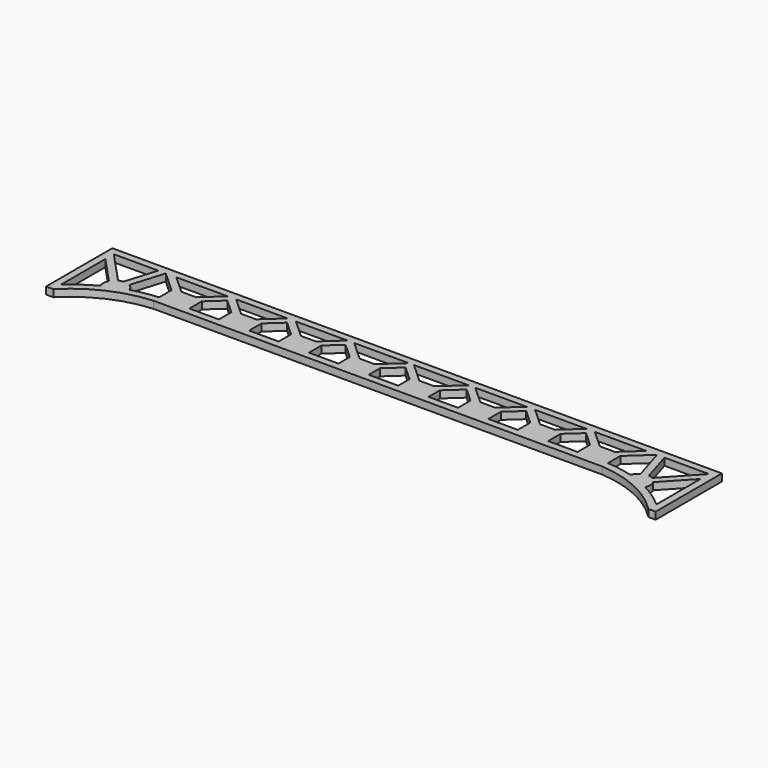
from build123d import *

# Parameters (mm, degrees)
F1_DEPTH = 1


# Not quite as in the source:
# - ends of sketch curves that miss each other by under 0.0002 mm in the source are joined


with BuildPart() as f1:
    # F0 (on Top) → F1 (new body)
    with BuildSketch(Plane.XY):
        with BuildLine():
            ThreePointArc((31.2898730428, -1.0903693776), (36.8162528215, -2.4992396802), (41.4861883055, -5.7729976987))
            Line((41.4861883055, -5.7729976987), (42.499983, -5.772998))
            Line((42.499983, -5.772998), (42.499983, 5.772998))
            Line((42.499983, 5.772998), (-42.499983, 5.772998))
            Line((-42.499983, 5.772998), (-42.499983, -5.772998))
            Line((-42.499983, -5.772998), (-41.486188, -5.772998))
            ThreePointArc((-41.486188, -5.772998), (-36.8162528215, -2.4992396802), (-31.2898730428, -1.0903693776))
            Line((-31.2898730428, -1.0903693776), (31.2898730428, -1.0903693776))
        make_face()
        with BuildLine():
            ThreePointArc((-37.980823226, -1.9562535657), (-39.8184929613, -3.0669655752), (-41.4999834083, -4.4023685483))
            Line((-41.4999834083, -4.4023685483), (-41.499983, 3.305772))
            Line((-41.499983, 3.305772), (-37.947737, -0.508143))
            ThreePointArc((-37.947737, -0.508143), (-38.1314028467, -1.2283801993), (-37.980823226, -1.9562535657))
        make_face(mode=Mode.SUBTRACT)
        with BuildLine():
            Line((41.499983, 3.305772), (41.499983, -4.402369))
            ThreePointArc((41.499983, -4.402369), (39.8184929613, -3.0669655752), (37.980823226, -1.9562535657))
            ThreePointArc((37.980823226, -1.9562535657), (38.1314028467, -1.2283801993), (37.9477363989, -0.5081433103))
            Line((37.9477363989, -0.5081433103), (41.499983, 3.305772))
        make_face(mode=Mode.SUBTRACT)
        with BuildLine():
            Line((-31.289873, 2.077969), (-31.289873, -0.09037))
            ThreePointArc((-31.289873, -0.09037), (-33.1211344425, -0.3089644519), (-34.9175362693, -0.7263880763))
            ThreePointArc((-34.9175362693, -0.7263880763), (-35.2042200678, -0.2151094555), (-35.6513559051, 0.1639211639))
            Line((-35.6513559051, 0.1639211639), (-34.24769, 4.772998))
            Line((-34.24769, 4.772998), (-31.289873, 2.077969))
        make_face(mode=Mode.SUBTRACT)
        with BuildLine():
            Line((-37.241042, 0.200331), (-41.499983, 4.772998))
            Line((-41.499983, 4.772998), (-35.293036, 4.772998))
            Line((-35.293036, 4.772998), (-36.631091, 0.379359))
            ThreePointArc((-36.631091, 0.379359), (-36.9447562748, 0.3194512642), (-37.241042, 0.200331))
        make_face(mode=Mode.SUBTRACT)
        Polygon((-22.953359, -0.09037), (-27.06573, -0.09037), (-27.06573, 2.077969), (-25.009544, 3.951473), (-22.953359, 2.077969), align=None, mode=Mode.SUBTRACT)
        Polygon((-14.616844, -0.09037), (-18.729215, -0.09037), (-18.729215, 2.077969), (-16.67303, 3.951473), (-14.616844, 2.077969), align=None, mode=Mode.SUBTRACT)
        Polygon((-6.280329, -0.09037), (-10.392701, -0.09037), (-10.392701, 2.077969), (-8.44277, 3.854658), (-6.280329, 1.884339), align=None, mode=Mode.SUBTRACT)
        Polygon((-25.584392, 4.772998), (-28.130887, 2.456623), (-30.224716, 2.456623), (-32.771212, 4.772998), align=None, mode=Mode.SUBTRACT)
        Polygon((-19.794373, 2.456623), (-21.888201, 2.456623), (-24.434697, 4.772998), (-17.247877, 4.772998), align=None, mode=Mode.SUBTRACT)
        Polygon((-11.457858, 2.456623), (-13.551687, 2.456623), (-16.098182, 4.772998), (-8.911362, 4.772998), align=None, mode=Mode.SUBTRACT)
        Polygon((-3.121343, 2.262993), (-5.215172, 2.262993), (-7.974534, 4.772998), (-0.361981, 4.772998), align=None, mode=Mode.SUBTRACT)
        Polygon((0, -0.09037), (-2.056186, -0.09037), (-2.056186, 1.884339), (0, 3.757843), (2.056186, 1.884339), (2.056186, -0.09037), align=None, mode=Mode.SUBTRACT)
        Polygon((10.392701, 2.077969), (10.392701, -0.09037), (6.280329, -0.09037), (6.280329, 1.884339), (8.44277, 3.854658), align=None, mode=Mode.SUBTRACT)
        Polygon((18.729215, 2.077969), (18.729215, -0.09037), (14.616844, -0.09037), (14.616844, 2.077969), (16.67303, 3.951473), align=None, mode=Mode.SUBTRACT)
        Polygon((27.06573, 2.077969), (27.06573, -0.09037), (22.953359, -0.09037), (22.953359, 2.077969), (25.009544, 3.951473), align=None, mode=Mode.SUBTRACT)
        with BuildLine():
            Line((31.289873, -0.09037), (31.289873, 2.077969))
            Line((31.289873, 2.077969), (34.24769, 4.772998))
            Line((34.24769, 4.772998), (35.651356, 0.163921))
            ThreePointArc((35.651356, 0.163921), (35.2042200678, -0.2151094555), (34.9175353631, -0.7263887799))
            ThreePointArc((34.9175353631, -0.7263887799), (33.1211344425, -0.3089644519), (31.289873, -0.09037))
        make_face(mode=Mode.SUBTRACT)
        with BuildLine():
            Line((35.293036, 4.772998), (41.499983, 4.772998))
            Line((41.499983, 4.772998), (37.241042, 0.200331))
            ThreePointArc((37.241042, 0.200331), (36.9447562748, 0.3194512642), (36.6310910035, 0.3793590379))
            Line((36.6310910035, 0.3793590379), (35.293036, 4.772998))
        make_face(mode=Mode.SUBTRACT)
        Polygon((7.974534, 4.772998), (5.215172, 2.262993), (3.121343, 2.262993), (0.361981, 4.772998), align=None, mode=Mode.SUBTRACT)
        Polygon((16.098182, 4.772998), (13.551687, 2.456623), (11.457858, 2.456623), (8.911362, 4.772998), align=None, mode=Mode.SUBTRACT)
        Polygon((24.434697, 4.772998), (21.888201, 2.456623), (19.794373, 2.456623), (17.247877, 4.772998), align=None, mode=Mode.SUBTRACT)
        Polygon((32.771212, 4.772998), (30.224716, 2.456623), (28.130887, 2.456623), (25.584392, 4.772998), align=None, mode=Mode.SUBTRACT)
    extrude(amount=F1_DEPTH)


solid = f1.part
